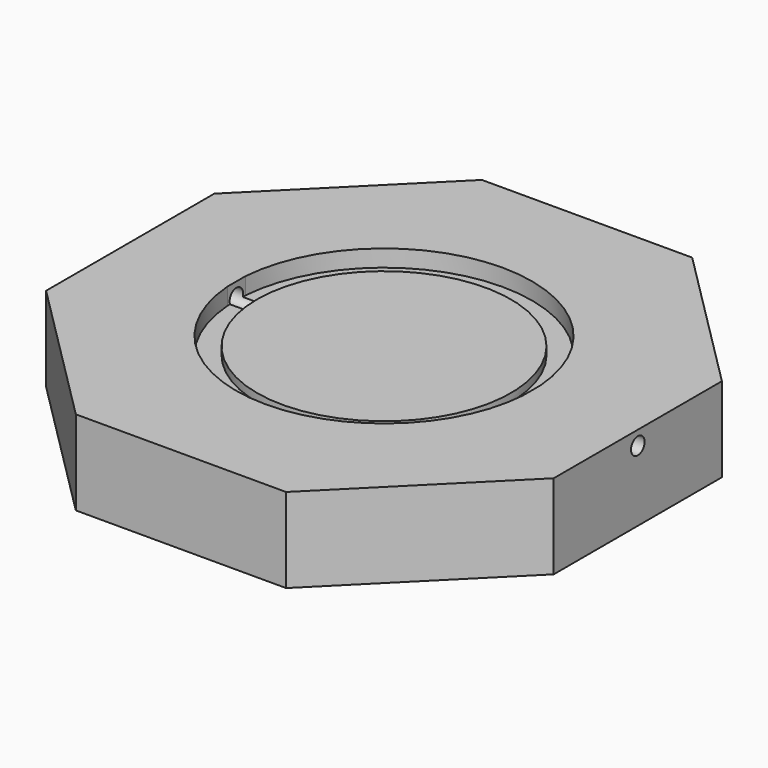
from build123d import *

# Parameters (mm, degrees)
F1_DEPTH       = 40
F2_R           = 22.5
F3_DEPTH       = 3
F5_DEPTH       = 25
F6_DEPTH       = 25
F7_DEPTH       = 25
F8_R           = 1.5
F9_DEPTH       = 110
F10_END_RADIUS = 22.5
F10_REACH      = 49.2436407871
F11_END_RADIUS = 22.5
F11_REACH      = 49.2436407871
F12_DEPTH      = 1.6


with BuildPart() as f1:
    # F0 (on Top) → F1 (new body)
    with BuildSketch(Plane.XY):
        Polygon((18.6396103068, 45), (-18.6396103068, 45), (-45, 18.6396103068), (-45, -18.6396103068), (-18.6396103068, -45), (18.6396103068, -45), (45, -18.6396103068), (45, 18.6396103068), align=None)
    extrude(amount=F1_DEPTH)

    # F2 (on face) → F3 (cut)
    with BuildSketch(Plane.XY.offset(40)):
        with BuildLine():
            Line((-26.1736986305, 2), (-26.1736986305, -2))
            ThreePointArc((-26.1736986305, -2), (0, -26.25), (26.1736986305, -2))
            Line((26.1736986305, -2), (26.1736986305, 2))
            ThreePointArc((26.1736986305, 2), (0, 26.25), (-26.1736986305, 2))
        make_face()
        Circle(F2_R, mode=Mode.SUBTRACT)
    extrude(amount=-F3_DEPTH, mode=Mode.SUBTRACT)

    # F4 (on face) → F5 (join)
    with BuildSketch(Plane.XY):
        Polygon((-18.6396103068, -45), (18.6396103068, -45), (45, -18.6396103068), (45, 18.6396103068), (18.6396103068, 45), (-18.6396103068, 45), (-45, 18.6396103068), (-45, -18.6396103068), align=None)
    extrude(amount=F5_DEPTH)

    # F0 (on Top) → F6 (join)
    with BuildSketch(Plane.XY):
        Polygon((18.6396103068, 45), (-18.6396103068, 45), (-45, 18.6396103068), (-45, -18.6396103068), (-18.6396103068, -45), (18.6396103068, -45), (45, -18.6396103068), (45, 18.6396103068), align=None)
    extrude(amount=F6_DEPTH)

    # F0 (on Top) → F7 (cut)
    with BuildSketch(Plane.XY):
        Polygon((18.6396103068, 45), (-18.6396103068, 45), (-45, 18.6396103068), (-45, -18.6396103068), (-18.6396103068, -45), (18.6396103068, -45), (45, -18.6396103068), (45, 18.6396103068), align=None)
    extrude(amount=F7_DEPTH, mode=Mode.SUBTRACT)

    # F8 (on Right) → F9 (cut, symmetric)
    with BuildSketch(Plane.YZ):
        with Locations((0, 37.5)):
            Circle(F8_R)
    extrude(amount=F9_DEPTH, both=True, mode=Mode.SUBTRACT)

    f10_end = (Plane.XY.offset(38.5) * Cylinder(F10_END_RADIUS, 354.8073942381, mode=Mode.PRIVATE)).faces().sort_by_distance((-22.5, 0, 39.3628971796))[0]
    # F8 (on Right) → F10 (join, up to the whole of a round face its end follows)
    with BuildSketch(Plane.YZ):
        with Locations((0, 37.5)):
            Circle(F8_R)
    f10_long = extrude(amount=F10_REACH, mode=Mode.PRIVATE)
    add(split(f10_long, bisect_by=f10_end, keep=Keep.BOTTOM, mode=Mode.PRIVATE))

    f11_end = (Plane.XY.offset(38.5) * Cylinder(F11_END_RADIUS, 354.8073942381, mode=Mode.PRIVATE)).faces().sort_by_distance((-22.5, 0, 39.3628971796))[0]
    # F8 (on Right) → F11 (join, up to the whole of a round face its end follows)
    with BuildSketch(Plane.YZ):
        with Locations((0, 37.5)):
            Circle(F8_R)
    f11_long = extrude(amount=-F11_REACH, mode=Mode.PRIVATE)
    add(split(f11_long, bisect_by=f11_end, keep=Keep.BOTTOM, mode=Mode.PRIVATE))

    # F12 (cut): a face of the model
    f12_faces = [f1.faces().sort_by_distance(p)[0] for p in [
        (0, 0, 40),
    ]]
    extrude(f12_faces, amount=-F12_DEPTH, mode=Mode.SUBTRACT)


solid = f1.part
